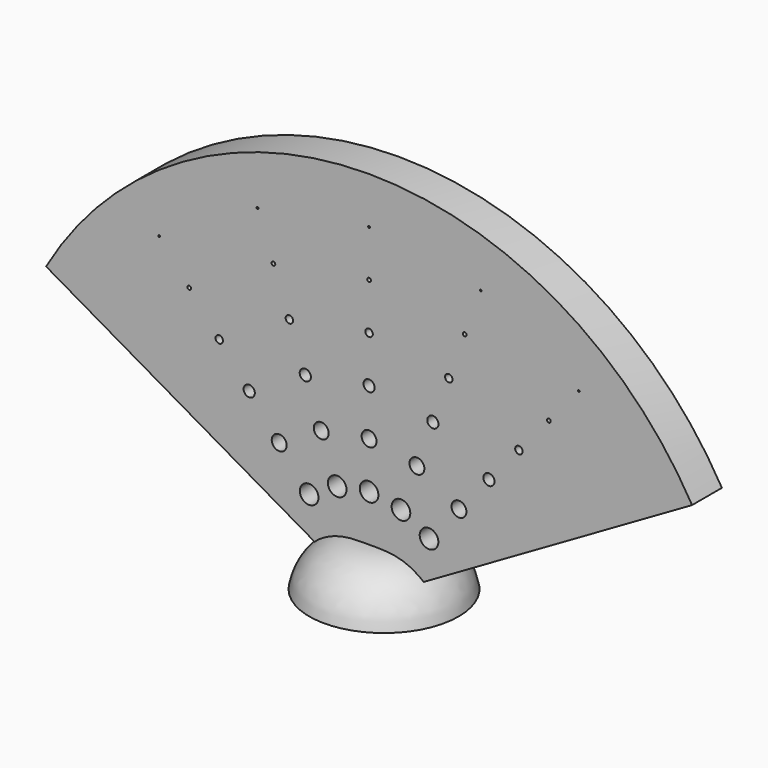
from build123d import *

# Parameters (mm, degrees)
F0_W          = 2
F0_H          = 20
F1_ANGLE_BACK = 60
F1_ANGLE      = 120
F2_R          = 4
F3_DEPTH      = 2.5
F5_R          = 0.5
F5_R_2        = 0.4
F5_R_3        = 0.3
F5_R_4        = 0.2
F5_R_5        = 0.1
F5_R_6        = 0.05
F6_DEPTH      = 25


# Not quite as in the source:
# - a fillet or chamfer that OpenCascade refuses, or shapes differently, is made with other operations: its cross-section is extruded or revolved along the edge and cut away or added


with BuildPart() as f1:
    # F0 (on Right) → F1 (revolve)
    with BuildSketch(Plane.YZ, mode=Mode.PRIVATE) as f1_sk:
        with Locations((1, 10)):
            Rectangle(F0_W, F0_H)
    revolve(f1_sk.sketch.rotate(Axis((0, 1, 0), (0, 1, 0)), -F1_ANGLE_BACK), axis=Axis((0, 1, 0), (0, 1, 0)), revolution_arc=F1_ANGLE)

    # F5 (on face) → F6 (cut)
    with BuildSketch(Plane.XZ):
        with Locations((0, 5)):
            Circle(F5_R)
        with Locations((0, 7.5)):
            Circle(F5_R_2)
        with Locations((0, 10)):
            Circle(F5_R_3)
        with Locations((0, 12.5)):
            Circle(F5_R_4)
        with Locations((0, 15)):
            Circle(F5_R_5)
        with Locations((0, 17.5)):
            Circle(F5_R_6)
        with Locations((-5.9853525082, 16.4446208638)):
            Circle(F5_R_6)
        with Locations((-5.1303021499, 14.0953893118)):
            Circle(F5_R_5)
        with Locations((-4.2752517916, 11.7461577598)):
            Circle(F5_R_4)
        with Locations((-3.4202014333, 9.3969262079)):
            Circle(F5_R_3)
        with Locations((-2.5651510749, 7.0476946559)):
            Circle(F5_R_2)
        with Locations((-1.7101007166, 4.6984631039)):
            Circle(F5_R)
        with Locations((-11.2487831695, 13.4057777546)):
            Circle(F5_R_6)
        with Locations((-9.6418141453, 11.4906666468)):
            Circle(F5_R_5)
        with Locations((-8.0348451211, 9.575555539)):
            Circle(F5_R_4)
        with Locations((-6.4278760969, 7.6604444312)):
            Circle(F5_R_3)
        with Locations((-4.8209070726, 5.7453333234)):
            Circle(F5_R_2)
        with Locations((-3.2139380484, 3.8302222156)):
            Circle(F5_R)
        with Locations((11.2487831695, 13.4057777546)):
            Circle(F5_R_6)
        with Locations((9.6418141453, 11.4906666468)):
            Circle(F5_R_5)
        with Locations((8.0348451211, 9.575555539)):
            Circle(F5_R_4)
        with Locations((6.4278760969, 7.6604444312)):
            Circle(F5_R_3)
        with Locations((4.8209070726, 5.7453333234)):
            Circle(F5_R_2)
        with Locations((3.2139380484, 3.8302222156)):
            Circle(F5_R)
        with Locations((5.9853525082, 16.4446208638)):
            Circle(F5_R_6)
        with Locations((5.1303021499, 14.0953893118)):
            Circle(F5_R_5)
        with Locations((4.2752517916, 11.7461577598)):
            Circle(F5_R_4)
        with Locations((3.4202014333, 9.3969262079)):
            Circle(F5_R_3)
        with Locations((2.5651510749, 7.0476946559)):
            Circle(F5_R_2)
        with Locations((1.7101007166, 4.6984631039)):
            Circle(F5_R)
    extrude(amount=-F6_DEPTH, mode=Mode.SUBTRACT)


with BuildPart() as f3:
    # F2 (on Top) → F3 (new body)
    with BuildSketch(Plane.XY):
        with Locations((0, 1)):
            Circle(F2_R)
    extrude(amount=F3_DEPTH)

    # F4: fillet of radius 3 on 1 edges, made by hand

    # F4_s1 → F4_t2 (revolve, cut)
    with BuildSketch(Plane.XZ.offset(-1)):
        with BuildLine():
            ThreePointArc((4, 0), (2.9784517816, 1.7912878475), (1.0419601084, 2.5))
            Line((1.0419601084, 2.5), (4, 2.5))
            Line((4, 2.5), (4, 0))
        make_face()
    revolve(axis=Axis((0, 1, 2.5), (0, 0, 1)), mode=Mode.SUBTRACT)


solid = Compound([f1.part, f3.part])
